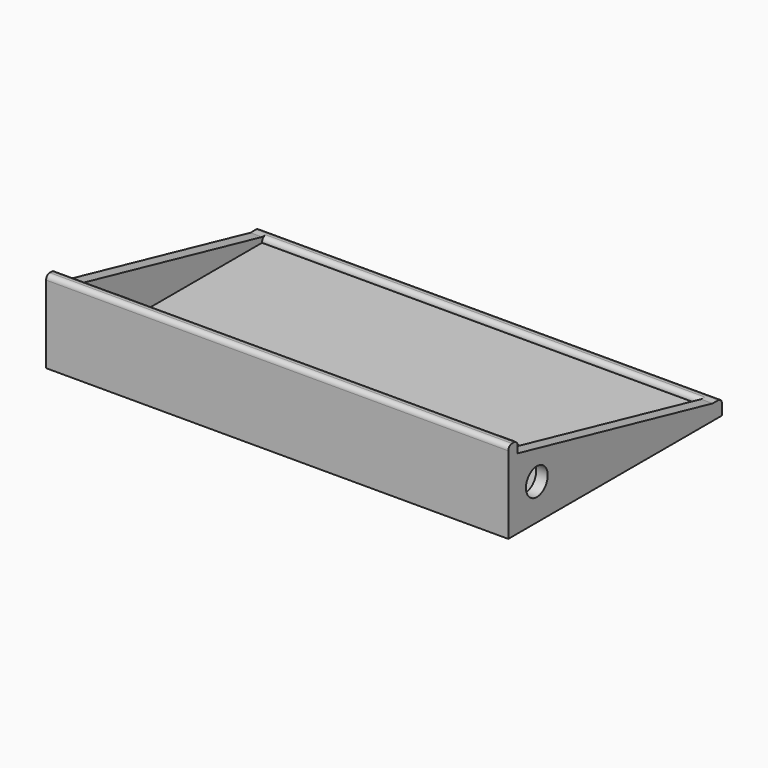
from build123d import *

# Parameters (mm, degrees)
F0_W          = 90
F0_H          = 52
F1_DEPTH      = 16
F3_DEPTH      = 1323
F0_W_2        = 2.3
F0_H_2        = 10
F4_DEPTH      = 12.2
F5_R          = 2.65
F6_DEPTH      = 100
F6_DEPTH_BACK = 25
F7_DEPTH      = 2
F8_R          = 7
F9_R          = 0.9


with BuildPart() as f1:
    # F0 (on Top) → F1 (new body)
    with BuildSketch(Plane.XY):
        Rectangle(F0_W, F0_H)
        Polygon((-42.75, 23.75), (42.75, 23.75), (42.75, -23.75), (38.55, -23.75), (36.25, -23.75), (-36.25, -23.75), (-38.55, -23.75), (-42.75, -23.75), align=None, mode=Mode.SUBTRACT)
    extrude(amount=F1_DEPTH)

    # F2 (on face) → F3 (cut)
    with BuildSketch(Plane(origin=(-45, 0, 0), x_dir=(0, -1, 0), z_dir=(-1, 0, 0))):
        Polygon((-26, 16), (-26, 3), (-23.75, 3), (23.75, 13.75), (23.75, 16), align=None)
    extrude(amount=-F3_DEPTH, mode=Mode.SUBTRACT)

    # F0 (on Top) → F4 (join)
    with BuildSketch(Plane.XY):
        with Locations((-37.4, -18.75)):
            Rectangle(F0_W_2, F0_H_2)
        with Locations((37.4, -18.75)):
            Rectangle(F0_W_2, F0_H_2)
    extrude(amount=F4_DEPTH)

    # F5 (on face) → F6 (cut, two sides)
    with BuildSketch(Plane(origin=(-38.55, 0, 0), x_dir=(0, -1, 0), z_dir=(-1, 0, 0))) as f6_sk:
        with Locations((19.05, 7)):
            Circle(F5_R)
    extrude(amount=-F6_DEPTH, mode=Mode.SUBTRACT)
    extrude(f6_sk.sketch, amount=F6_DEPTH_BACK, mode=Mode.SUBTRACT)

    # F0 (on Top) → F7 (join)
    with BuildSketch(Plane.XY):
        Rectangle(F0_W, F0_H)
        Polygon((-42.75, 23.75), (42.75, 23.75), (42.75, -23.75), (38.55, -23.75), (36.25, -23.75), (-36.25, -23.75), (-38.55, -23.75), (-42.75, -23.75), align=None, mode=Mode.SUBTRACT)
        Polygon((42.75, -23.75), (42.75, 23.75), (-42.75, 23.75), (-42.75, -23.75), (-38.55, -23.75), (-38.55, -13.75), (-36.25, -13.75), (-36.25, -23.75), (36.25, -23.75), (36.25, -13.75), (38.55, -13.75), (38.55, -23.75), align=None)
    extrude(amount=F7_DEPTH)

    # F8
    f8_edges = [f1.edges().sort_by_distance(p)[0] for p in [
        (-37.4, -13.75, 12.2),
        (37.4, -13.75, 12.2),
    ]]
    fillet(f8_edges, radius=F8_R)

    # F9
    f9_edges = [f1.edges().sort_by_distance(p)[0] for p in [
        (0, -26, 16),
        (0, -23.75, 16),
        (0, 23.75, 3),
        (0, 26, 3),
    ]]
    fillet(f9_edges, radius=F9_R)


solid = f1.part
